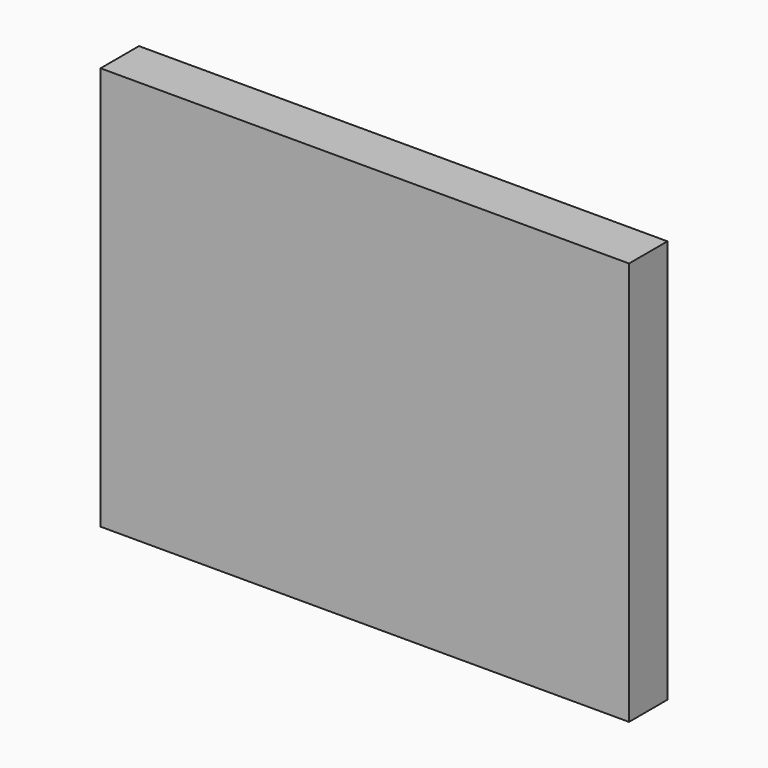
from build123d import *

# Parameters (mm, degrees)
F1_DEPTH = 3.175


# Not quite as in the source:
# - a feature names something its author has since deleted; it is built from what else it names


with BuildPart() as f1:
    # F0 (on Front) → F1 (new body)
    with BuildSketch(Plane.XZ):
        Polygon((19.05, 11.43), (19.05, 38.1), (-15.875, 38.1), (-15.875, 29.21), (-15.875, 20.32), (-15.875, 11.43), align=None)
    extrude(amount=F1_DEPTH)


solid = f1.part
